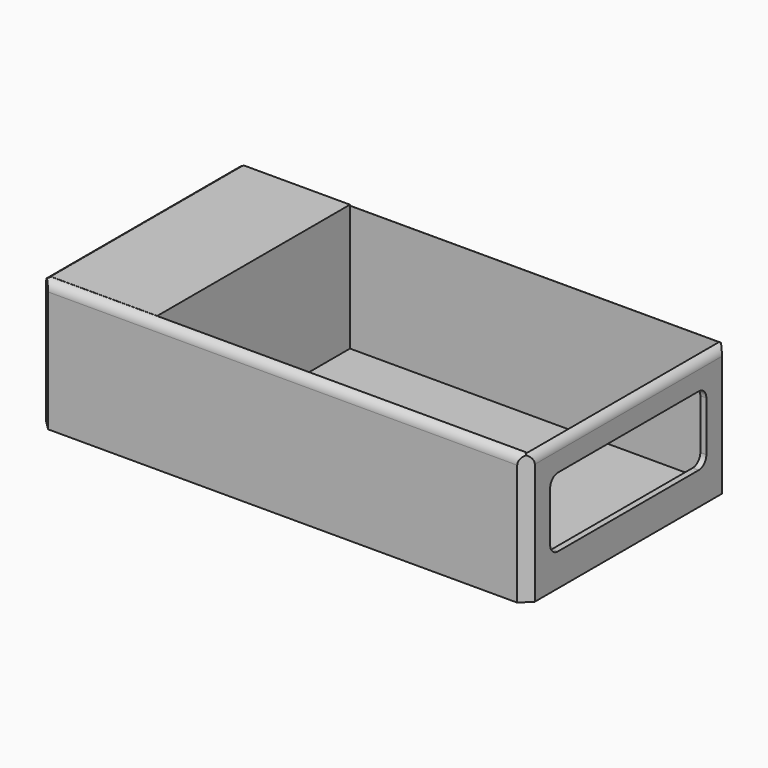
from build123d import *

# Parameters (mm, degrees)
F0_W        = 250.7199645042
F0_H        = 67.0627206564
F1_DEPTH    = 130
F2_W        = 244.152829051
F2_H        = 123.597616097
F3_DEPTH    = 65.1
F4_SIZE     = 5
F5_T1_DEPTH = 145
F5_T3_DEPTH = 265.7199645042
F6_W        = 100.1766752452
F6_H        = 35.6183759868
F7_DEPTH    = 25
F8_R        = 5
F9_W        = 54.5746013522
F9_H        = 123.597616097
F10_DEPTH   = 65


# Not quite as in the source:
# - a fillet or chamfer that OpenCascade refuses, or shapes differently, is made with other operations: its cross-section is extruded or revolved along the edge and cut away or added


with BuildPart() as f1:
    # F0 (on Front) → F1 (new body)
    with BuildSketch(Plane.XZ):
        Rectangle(F0_W, F0_H)
    extrude(amount=-F1_DEPTH)

    # F2 (on face) → F3 (cut)
    with BuildSketch(Plane.XY.offset(33.5313603282)):
        with Locations((0.1901462674, 65.5300348299)):
            Rectangle(F2_W, F2_H)
    extrude(amount=-F3_DEPTH, mode=Mode.SUBTRACT)

    # F4
    f4_edges = [f1.edges().sort_by_distance(p)[0] for p in [
        (-125.359982, 0, 0),
        (-125.359982, 130, 0),
        (125.359982, 130, 0),
        (125.359982, 0, 0),
    ]]
    chamfer(f4_edges, length=F4_SIZE)

    # F5: fillet of radius 5 on 4 edges, made by hand

    # F5_s2 → F5_t1 (cut)
    with BuildSketch(Plane.XZ.offset(-137.5)):
        with BuildLine():
            ThreePointArc((-125.3599822521, 28.5313603282), (-123.8955161581, 32.0668942341), (-120.3599822521, 33.5313603282))
            Line((-120.3599822521, 33.5313603282), (-125.3599822521, 33.5313603282))
            Line((-125.3599822521, 33.5313603282), (-125.3599822521, 28.5313603282))
        make_face()
        with BuildLine():
            ThreePointArc((125.3599822521, 28.5313603282), (123.8955161581, 32.0668942341), (120.3599822521, 33.5313603282))
            Line((120.3599822521, 33.5313603282), (125.3599822521, 33.5313603282))
            Line((125.3599822521, 33.5313603282), (125.3599822521, 28.5313603282))
        make_face()
    extrude(amount=F5_T1_DEPTH, mode=Mode.SUBTRACT)

    # F5_s4 → F5_t3 (cut)
    with BuildSketch(Plane.YZ.offset(-132.8599822521)):
        with BuildLine():
            ThreePointArc((130, 28.5313603282), (128.5355339059, 32.0668942341), (125, 33.5313603282))
            Line((125, 33.5313603282), (130, 33.5313603282))
            Line((130, 33.5313603282), (130, 28.5313603282))
        make_face()
        with BuildLine():
            ThreePointArc((0, 28.5313603282), (1.4644660941, 32.0668942341), (5, 33.5313603282))
            Line((5, 33.5313603282), (0, 33.5313603282))
            Line((0, 33.5313603282), (0, 28.5313603282))
        make_face()
    extrude(amount=F5_T3_DEPTH, mode=Mode.SUBTRACT)

    # F6 (on face) → F7 (cut)
    with BuildSketch(Plane.YZ.offset(125.3599822521)):
        with Locations((64.9271169677, 0.9739398956)):
            Rectangle(F6_W, F6_H)
    extrude(amount=-F7_DEPTH, mode=Mode.SUBTRACT)

    # F8
    f8_edges = [f1.edges().sort_by_distance(p)[0] for p in [
        (123.813272, 14.838779, 18.783128),
        (123.813272, 115.015455, 18.783128),
        (123.813272, 115.015455, -16.835248),
        (123.813272, 14.838779, -16.835248),
    ]]
    fillet(f8_edges, radius=F8_R)


with BuildPart() as f10:
    # F9 (on face) → F10 (new body)
    with BuildSketch(Plane.XY.offset(-31.5686396718)):
        with Locations((-94.598967582, 65.5300348299)):
            Rectangle(F9_W, F9_H)
    extrude(amount=F10_DEPTH)


solid = Compound([f1.part, f10.part])
